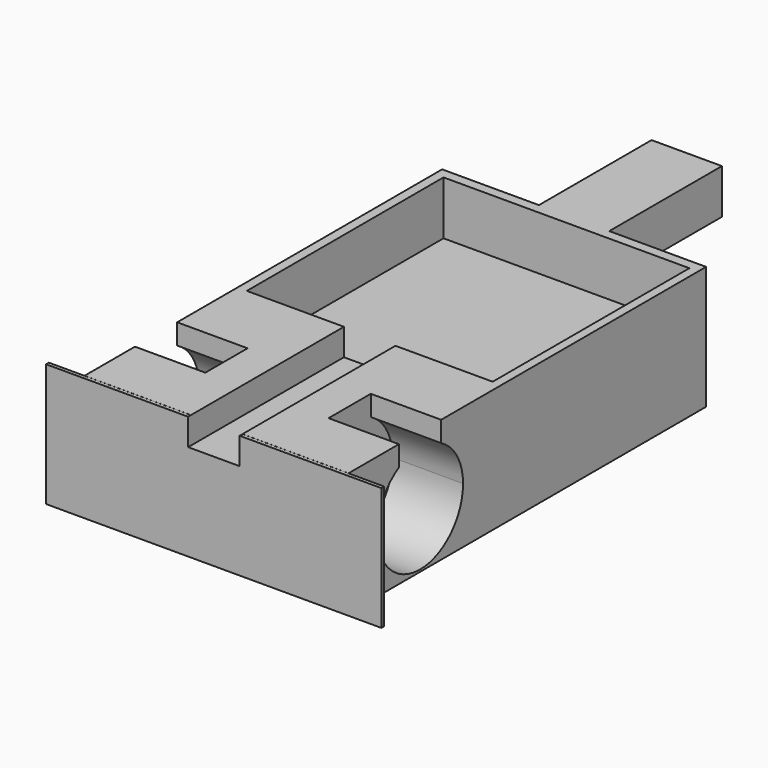
from build123d import *

# Parameters (mm, degrees)
F0_W      = 75
F0_H      = 35
F1_DEPTH  = 127
F3_DEPTH  = 20
F5_W      = 19.9898
F5_H      = 12.7
F6_DEPTH  = 40
F7_W      = 69.85
F7_H      = 69.85
F8_DEPTH  = 15.24
F9_W      = 95.2556729317
F9_H      = 34.9658876657
F10_DEPTH = 1
F11_W     = 14.6372080781
F11_H     = 57.15
F12_DEPTH = 7.62
F13_W     = 30.48
F13_H     = 93.98
F14_DEPTH = 15.24
F15_W     = 15.2369
F15_H     = 6.35
F16_DEPTH = 15.24


# Not quite as in the source:
# - a feature names something its author has since deleted; it is built from what else it names


with BuildPart() as f1:
    # F0 (on Front) → F1 (new body)
    with BuildSketch(Plane.XZ):
        Rectangle(F0_W, F0_H)
    extrude(amount=-F1_DEPTH)

    # F2 (on face) → F3 (cut)
    with BuildSketch(Plane.YZ.offset(37.5)):
        with BuildLine():
            ThreePointArc((17.9, 11.676062799), (25.4, 13.6444626123), (32.9, 11.676062799))
            Line((32.9, 11.676062799), (32.9, 17.5))
            Line((32.9, 17.5), (17.9, 17.5))
            Line((17.9, 17.5), (17.9, 11.676062799))
        make_face()
        with BuildLine():
            Line((32.9, 9.7889252245), (32.9, 11.676062799))
            ThreePointArc((32.9, 11.676062799), (25.4, 13.6444626123), (17.9, 11.676062799))
            Line((17.9, 11.676062799), (17.9, 9.7889252245))
            Line((17.9, 9.7889252245), (32.9, 9.7889252245))
        make_face()
        with BuildLine():
            ThreePointArc((17.9, 11.676062799), (17.6959593413, -14.8149434406), (40.672455682, -1.6279930697))
            ThreePointArc((40.672455682, -1.6279930697), (38.586950371, 6.076047589), (32.9, 11.676062799))
            Line((32.9, 11.676062799), (32.9, 9.7889252245))
            Line((32.9, 9.7889252245), (17.9, 9.7889252245))
            Line((17.9, 9.7889252245), (17.9, 11.676062799))
        make_face()
    extrude(amount=-F3_DEPTH, mode=Mode.SUBTRACT)

    # F4: F1 across plane


with BuildPart() as f1_1:
    add(f1.part)
    add(f1.part.mirror(Plane.YZ), mode=Mode.INTERSECT)

    # F5 (on face) → F6 (join)
    with BuildSketch(Plane(origin=(0, 127, 0), x_dir=(-1, 0, 0), z_dir=(0, 1, 0))):
        with Locations((0.0051, 11.15)):
            Rectangle(F5_W, F5_H)
    extrude(amount=F6_DEPTH)

    # F7 (on face) → F8 (cut)
    with BuildSketch(Plane.XY.offset(17.5)):
        with Locations((0.075, 89.2494911432)):
            Rectangle(F7_W, F7_H)
    extrude(amount=-F8_DEPTH, mode=Mode.SUBTRACT)

    # F9 (on Front) → F10 (join)
    with BuildSketch(Plane.XZ):
        Rectangle(F9_W, F9_H)
    extrude(amount=F10_DEPTH)

    # F11 (on face) → F12 (cut)
    with BuildSketch(Plane.XY.offset(17.5)):
        with Locations((0.0553701539, 27.575)):
            Rectangle(F11_W, F11_H)
    extrude(amount=-F12_DEPTH, mode=Mode.SUBTRACT)

    # F13 (on face) → F14 (cut)
    with BuildSketch(Plane(origin=(0, 0, -17.5), x_dir=(1, 0, 0), z_dir=(0, 0, -1))):
        with Locations((0.0031, -73.66)):
            Rectangle(F13_W, F13_H)
    extrude(amount=-F14_DEPTH, mode=Mode.SUBTRACT)

    # F15 (on face) → F16 (cut)
    with BuildSketch(Plane(origin=(0, 0, -17.5), x_dir=(1, 0, 0), z_dir=(0, 0, -1))):
        with Locations((-7.61845, -123.825)):
            Rectangle(F15_W, F15_H)
    extrude(amount=-F16_DEPTH, mode=Mode.SUBTRACT)


solid = f1_1.part
